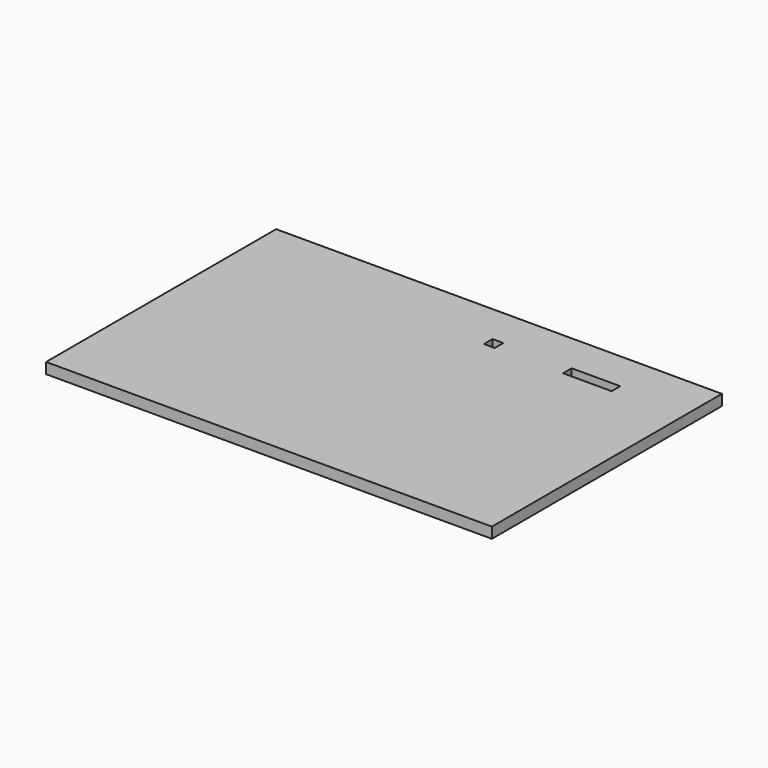
from build123d import *

# Parameters (mm, degrees)
F0_W     = 124
F0_H     = 80
F0_W_2   = 3
F0_H_2   = 3
F0_W_3   = 13.5
F1_DEPTH = 3


# Not quite as in the source:
# - a feature names something its author has since deleted; it is built from what else it names


with BuildPart() as f1:
    # F0 (on Top) → F1 (new body)
    with BuildSketch(Plane.XY):
        with Locations((-6.0411174464, 30)):
            Rectangle(F0_W, F0_H)
        with Locations((2.4588825536, 57.5)):
            Rectangle(F0_W_2, F0_H_2, mode=Mode.SUBTRACT)
        with Locations((29.7163994456, 57.5)):
            Rectangle(F0_W_3, F0_H_2, mode=Mode.SUBTRACT)
    extrude(amount=F1_DEPTH)


solid = f1.part
